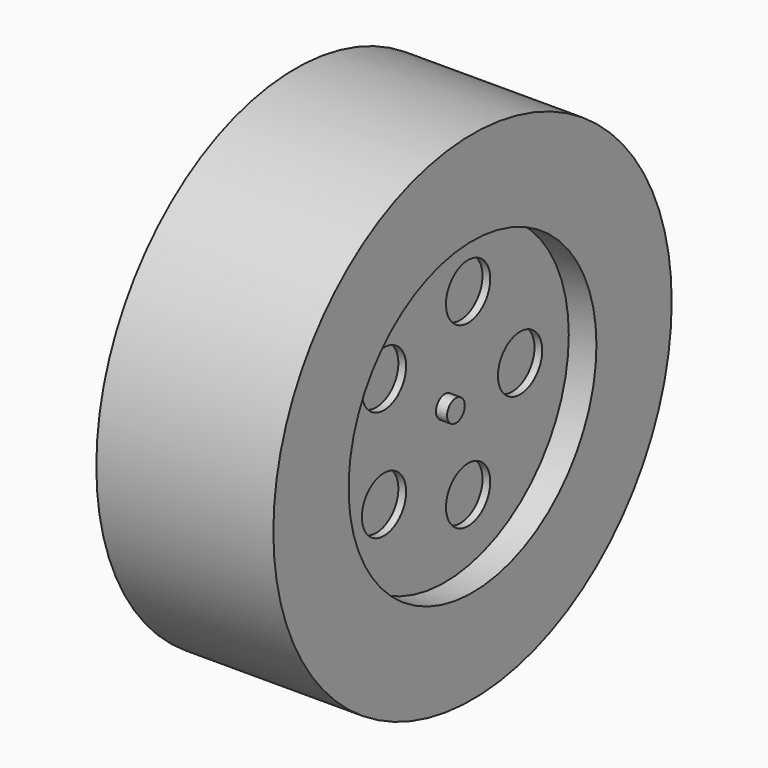
from build123d import *

# Parameters (mm, degrees)
F3_R            = 225
F4_DEPTH        = 160
F5_R            = 140
F6_DEPTH        = 25
F7_R            = 25
F8_DEPTH        = 7
F8_COPIES_COUNT = 5
F9_R            = 10
F10_DEPTH       = 10


# Not quite as in the source:
# - a pattern or mirror of a feature is missing from the dataset's text; its kind, count and spacing are read off the source's solid


with BuildPart() as f4:
    # F3 (on Right) → F4 (new body)
    with BuildSketch(Plane.YZ):
        Circle(F3_R)
    extrude(amount=F4_DEPTH)

    # F5 (on face) → F6 (cut)
    with BuildSketch(Plane.YZ.offset(160)):
        Circle(F5_R)
    extrude(amount=-F6_DEPTH, mode=Mode.SUBTRACT)

    # F7 (on face) → F8 (cut)
    with BuildSketch(Plane.YZ.offset(135)):
        with Locations((85, 0)):
            Circle(F7_R)
    f8 = extrude(amount=-F8_DEPTH, mode=Mode.SUBTRACT)

    # F8_copies: F8 ×5 about axis
    f8_copies_axis = Axis((0, 0, 0), (1, 0, 0))
    for i in range(1, F8_COPIES_COUNT):
        add(f8.rotate(f8_copies_axis, i * 360 / F8_COPIES_COUNT), mode=Mode.SUBTRACT)

    # F9 (on face) → F10 (join)
    with BuildSketch(Plane.YZ.offset(135)):
        Circle(F9_R)
    extrude(amount=F10_DEPTH)


solid = f4.part
